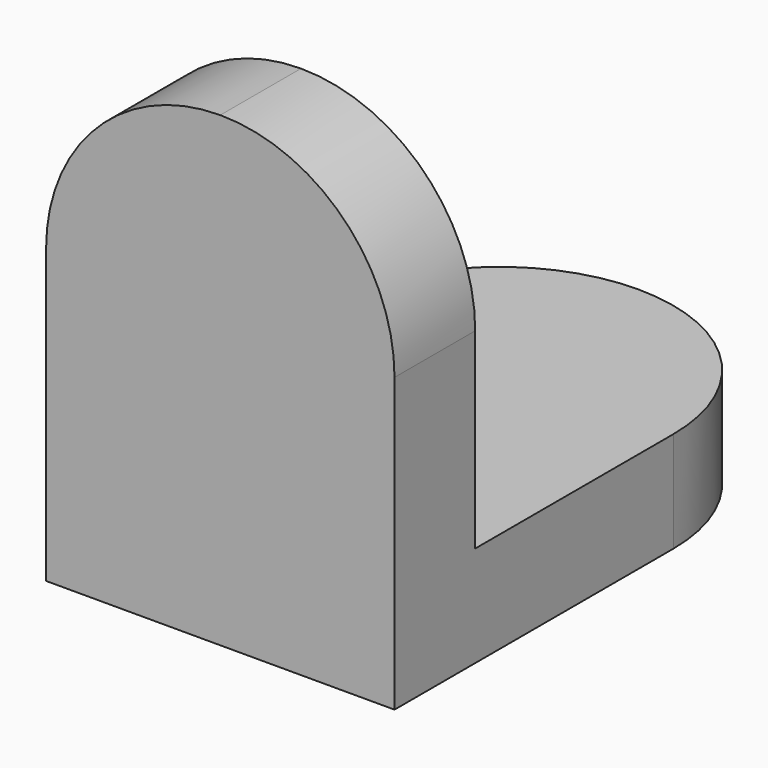
from build123d import *

# Parameters (mm, degrees)
F1_DEPTH = 38
F2_R     = 18.99999
F3_R     = 18.99999


# Not quite as in the source:
# - a fillet or chamfer is up to 0.001 mm smaller than in the source, because OpenCascade refuses the exact size


with BuildPart() as f1:
    # F0 (on Right) → F1 (new body)
    with BuildSketch(Plane.YZ):
        Polygon((-6.256232895, 31.9699999726), (-17.256232895, 31.9699999726), (-17.256232895, -18.9337489045), (39.743767105, -18.9337489045), (39.743767105, -7.9337489045), (-6.256232895, -7.9337489045), align=None)
    extrude(amount=F1_DEPTH)

    # F2 (radius 19 in the source; OpenCascade refuses exactly that, so slightly less here)
    f2_edges = [f1.edges().sort_by_distance(p)[0] for p in [
        (38, -11.756233, 31.97),
        (0, -11.756233, 31.97),
    ]]
    fillet(f2_edges, radius=F2_R)

    # F3 (radius 19 in the source; OpenCascade refuses exactly that, so slightly less here)
    f3_edges = [f1.edges().sort_by_distance(p)[0] for p in [
        (38, 39.743767, -13.433749),
        (0, 39.743767, -13.433749),
    ]]
    fillet(f3_edges, radius=F3_R)


solid = f1.part
